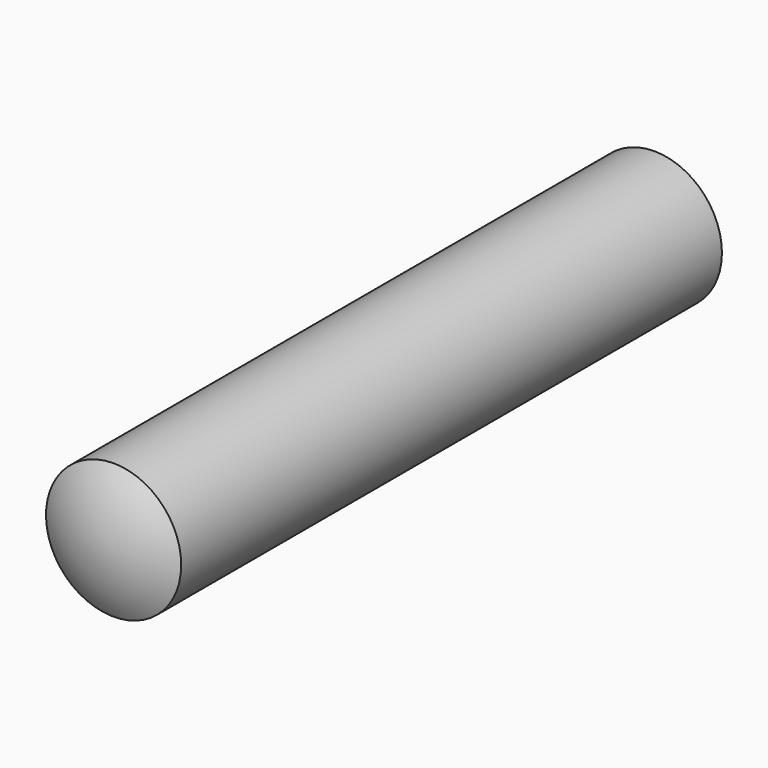
from build123d import *

# Parameters (mm, degrees)
F0_R          = 6
F1_DEPTH      = 30
F1_DEPTH_BACK = 30


# Not quite as in the source:
# - a pattern or mirror of a feature is missing from the dataset's text; its kind, count and spacing are read off the source's solid


with BuildPart() as f1:
    # F0 (on Front) → F1 (new body, two sides)
    with BuildSketch(Plane.XZ) as f1_sk:
        Circle(F0_R)
    extrude(amount=F1_DEPTH)
    extrude(f1_sk.sketch, amount=-F1_DEPTH_BACK)

    # F2 (on Right) → F3 (revolve)
    with BuildSketch(Plane.YZ):
        with BuildLine():
            Line((-31.8, 0), (-30, 0))
            Line((-30, 0), (-30, 6))
            ThreePointArc((-30, 6), (-31.3403065089, 3.1320919527), (-31.8, 0))
        make_face()
    f3 = revolve(axis=Axis((0, 0, 0), (0, 1, 0)))

    # F3_copies: F3 across plane
    add(f3.mirror(Plane.ZX))


solid = f1.part
